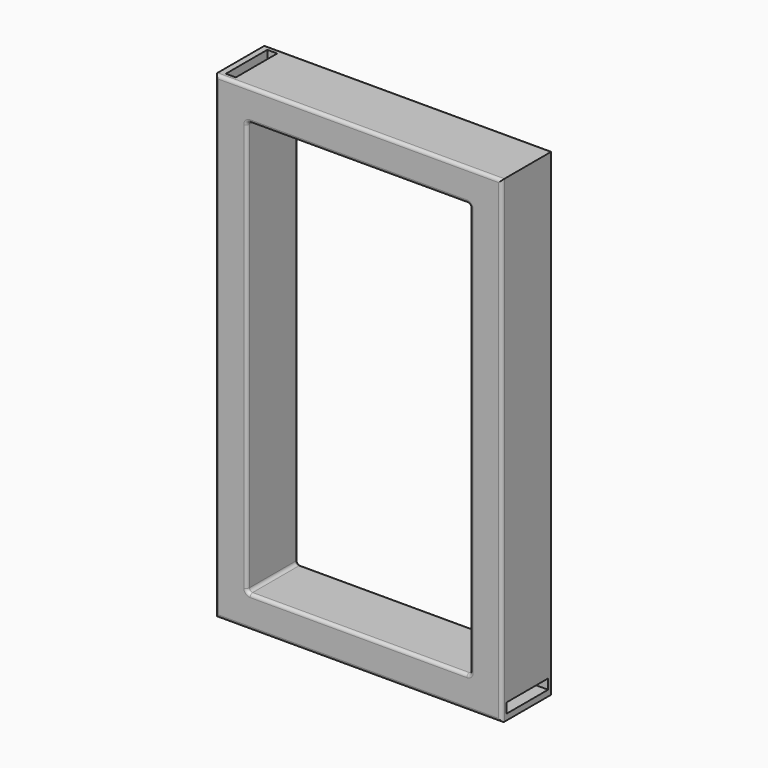
from build123d import *

# Parameters (mm, degrees)
F1_W     = 101.6
F1_H     = 50.8
F1_W_2   = 82.55
F1_H_2   = 34.8846255165
F4_W     = 50.8
F4_H     = 101.6
F4_W_2   = 31.75
F4_H_2   = 82.55
F6_DEPTH = 50.8
F7_F1_R  = 5.08
F7_F2_R  = 5.08
F8_R     = 5.08


with BuildPart() as f2:
    # F2: sweep along a path in F0
    with BuildLine(Plane.XZ) as f2_path:
        Line((0, 0), (406.4, 0))
        Line((406.4, 0), (406.4, -711.2))
    # F1 (on Right) → F2 (sweep)
    with BuildSketch(Plane.YZ):
        Rectangle(F1_W, F1_H)
        Rectangle(F1_W_2, F1_H_2, mode=Mode.SUBTRACT)
    sweep(path=f2_path.line, transition=Transition.RIGHT)

    # F5: sweep along a path in F0
    with BuildLine(Plane.XZ) as f5_path:
        Line((0, 0), (0, -711.2))
        Line((0, -711.2), (406.4, -711.2))
    # F4 (on offset) → F5 (sweep)
    with BuildSketch(Plane.XY.offset(25.4)):
        Rectangle(F4_W, F4_H)
        Rectangle(F4_W_2, F4_H_2, mode=Mode.SUBTRACT)
    sweep(path=f5_path.line, transition=Transition.RIGHT)

    # F6 (add): a face of the model
    f6_faces = [f2.faces().sort_by_distance(p)[0] for p in [
        (381, 0, -728.8136904762),
    ]]
    extrude(f6_faces, amount=F6_DEPTH)

    # F7: fillet of radius 5.08 on 6 edges, made by hand

    # F7_f1
    f7_f1_edges = [f2.edges().sort_by_distance(p)[0] for p in [
        (381, 0, -685.8),
        (25.4, 0, -685.8),
        (25.4, 0, -25.4),
        (381, 0, -25.4),
    ]]
    fillet(f7_f1_edges, radius=F7_F1_R)

    # F7_f2
    f7_f2_edges = [f2.edges().sort_by_distance(p)[0] for p in [
        (203.2, -50.8, -25.4),
        (25.4, 50.8, -355.6),
        (26.8878975516, 50.8, -26.8878975516),
        (26.8878975516, 50.8, -684.3121024484),
        (26.8878975516, -50.8, -26.8878975516),
        (379.5121024484, -50.8, -26.8878975516),
    ]]
    fillet(f7_f2_edges, radius=F7_F2_R)

    # F8
    f8_edges = [f2.edges().sort_by_distance(p)[0] for p in [
        (203.2, -50.8, 25.4),
        (-25.4, -50.8, -355.6),
        (431.8, -50.8, -355.6),
        (203.2, -50.8, -736.6),
        (-25.4, 50.8, -355.6),
        (203.2, 50.8, -736.6),
        (431.8, 50.8, -355.6),
        (203.2, 50.8, 25.4),
    ]]
    fillet(f8_edges, radius=F8_R)


solid = f2.part
